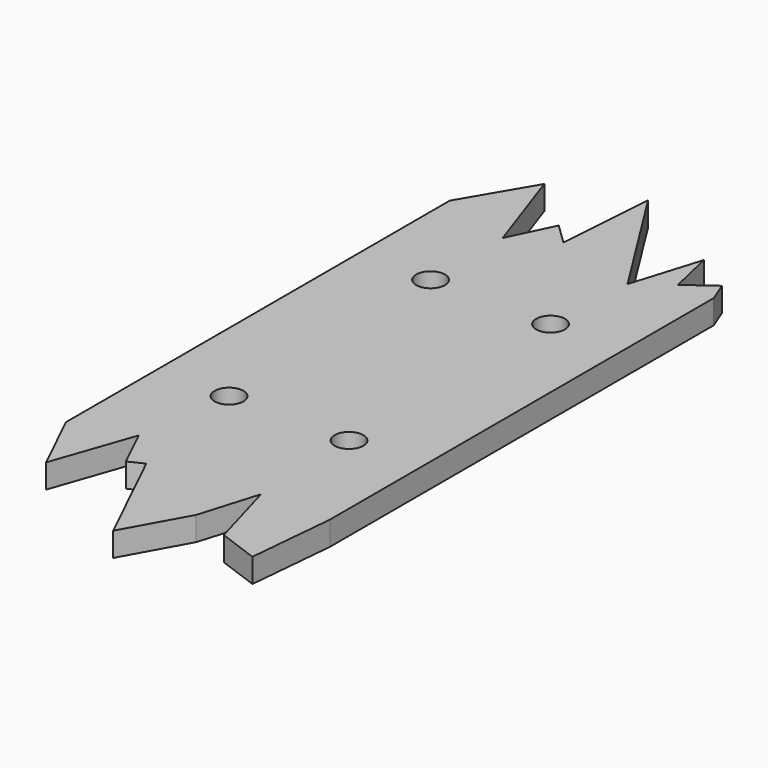
from build123d import *

# Parameters (mm, degrees)
F1_DEPTH = 10
F2_R     = 6
F3_DEPTH = 10.001


# Not quite as in the source:
# - a pattern or mirror of a feature is missing from the dataset's text; its kind, count and spacing are read off the source's solid


with BuildPart() as f1:
    # F0 (on Top) → F1 (new body)
    with BuildSketch(Plane.XY):
        Polygon((-55, 100), (-55, -100), (-42.3276498914, -126.1771321297), (-30.6749343872, -92.5011336803), (-22.4767297883, -109.4360733855), (-16.331512481, -106.4611735826), (4.8077032396, -150.1282154724), (18.9439784735, -124.5355084538), (26.3201091439, -100), (34.8079055548, -130.0195604563), (51.677390933, -136.1848264933), (55, -100), (55, 100), (51.677390933, 108.4323301911), (40.0880090892, 100), (35.7317700982, 118.9388260245), (26.9271209836, 90.1910439134), (-4.7420188785, 140.4679864645), (-7.6231127605, 100), (-16.331512481, 108.4323301911), (-25.1079257578, 90.1910439134), (-38.313575089, 128.3779740334), align=None)
    extrude(amount=F1_DEPTH)

    # F2 (on face) → F3 (cut, through all)
    with BuildSketch(Plane.XY.offset(10)):
        with Locations((-25, 52.5)):
            Circle(F2_R)
    f3 = extrude(amount=-F3_DEPTH, mode=Mode.SUBTRACT)

    # F3_copies: F3 across plane
    add(f3.mirror(Plane(origin=(0, 0, 0), x_dir=(0, 0, -1), z_dir=(0, -1, 0))), mode=Mode.SUBTRACT)

    # F3_copies1: F3 across plane
    add(f3.mirror(Plane(origin=(0, 0, 0), x_dir=(0, 0, 1), z_dir=(1, 0, 0))), mode=Mode.SUBTRACT)

    # F3_copies2: F3 across plane
    add(f3.mirror(Plane(origin=(0, 0, 0), x_dir=(-0.9028605188, -0.4299335804, 0), z_dir=(0.4299335804, -0.9028605188, 0))), mode=Mode.SUBTRACT)


solid = f1.part
